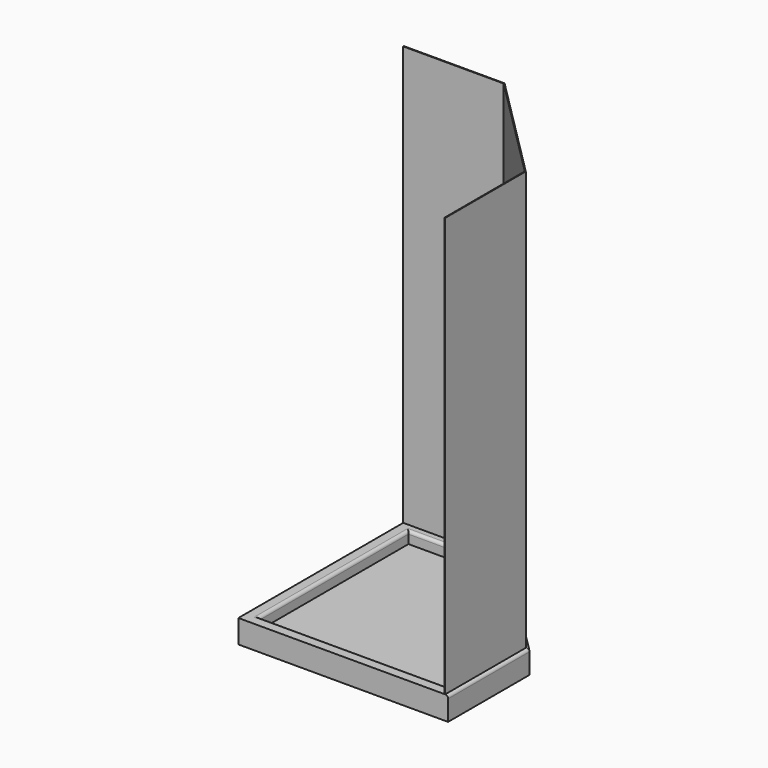
from build123d import *

# Parameters (mm, degrees)
F1_DEPTH     = 101.6
F2_T         = -50.8
F3_T1_DEPTH  = 508
F3_T3_DEPTH  = 728.0389529591
F3_T5_DEPTH  = 508
F3_T7_DEPTH  = 812.8
F3_T9_DEPTH  = 812.8
F3_T14_DEPTH = 685.954855022
F3_T20_DEPTH = 404.4079510314
F3_T25_DEPTH = 404.4079510314
F3_T31_DEPTH = 685.954855022
F3_T35_DEPTH = 404.4079510314
F3_T42_DEPTH = 404.4079510314
F3_T46_DEPTH = 685.954855022
F3_T53_DEPTH = 436.1579510314
F3_T57_DEPTH = 844.55
F3_T64_DEPTH = 844.55
F3_T68_DEPTH = 844.55
F3_T75_DEPTH = 844.55
F3_T79_DEPTH = 436.1579510314
F5_DEPTH     = 1828.8


# Not quite as in the source:
# - a fillet or chamfer that OpenCascade refuses, or shapes differently, is made with other operations: its cross-section is extruded or revolved along the edge and cut away or added


with BuildPart() as f1:
    # F0 (on Top) → F1 (new body)
    with BuildSketch(Plane.XY):
        Polygon((0, 914.4), (0, 0), (914.4, 0), (914.4, 444.5), (444.5, 914.4), align=None)
    extrude(amount=F1_DEPTH)

    # F2
    f2_openings = [f1.faces().sort_by_distance(p)[0] for p in [
        (411.47539, 411.47539, 101.6),
    ]]
    offset(amount=F2_T, openings=f2_openings)

    # F3: fillet of radius 12.7 on 11 edges, made by hand

    # F3_s2 → F3_t1 (cut)
    with BuildSketch(Plane.XZ.offset(-476.25)):
        with BuildLine():
            ThreePointArc((914.4, 88.9), (910.6802561211, 97.8802561211), (901.7, 101.6))
            Line((901.7, 101.6), (914.4, 101.6))
            Line((914.4, 101.6), (914.4, 88.9))
        make_face()
    extrude(amount=F3_T1_DEPTH, mode=Mode.SUBTRACT)

    # F3_s4 → F3_t3 (cut)
    with BuildSketch(Plane(origin=(257.4006403027, -257.4006403027, 0), x_dir=(0, 0, 1), z_dir=(-0.7071067812, 0.7071067812, 0))):
        with BuildLine():
            ThreePointArc((88.9, 960.8874049544), (97.8802561211, 957.1676610755), (101.6, 948.1874049544))
            Line((101.6, 948.1874049544), (101.6, 960.8874049544))
            Line((101.6, 960.8874049544), (88.9, 960.8874049544))
        make_face()
    extrude(amount=F3_T3_DEPTH, mode=Mode.SUBTRACT)

    # F3_s6 → F3_t5 (cut)
    with BuildSketch(Plane.YZ.offset(-31.75)):
        with BuildLine():
            ThreePointArc((914.4, 88.9), (910.6802561211, 97.8802561211), (901.7, 101.6))
            Line((901.7, 101.6), (914.4, 101.6))
            Line((914.4, 101.6), (914.4, 88.9))
        make_face()
    extrude(amount=F3_T5_DEPTH, mode=Mode.SUBTRACT)

    # F3_s8 → F3_t7 (cut)
    with BuildSketch(Plane.YZ.offset(50.8)):
        with BuildLine():
            ThreePointArc((38.1, 101.6), (47.0802561211, 97.8802561211), (50.8, 88.9))
            Line((50.8, 88.9), (50.8, 101.6))
            Line((50.8, 101.6), (38.1, 101.6))
        make_face()
    extrude(amount=F3_T7_DEPTH, mode=Mode.SUBTRACT)

    # F3_s10 → F3_t9 (cut)
    with BuildSketch(Plane.XZ.offset(-863.6)):
        with BuildLine():
            ThreePointArc((38.1, 101.6), (47.0802561211, 97.8802561211), (50.8, 88.9))
            Line((50.8, 88.9), (50.8, 101.6))
            Line((50.8, 101.6), (38.1, 101.6))
        make_face()
    extrude(amount=F3_T9_DEPTH, mode=Mode.SUBTRACT)


with BuildPart() as f3_tool12:
    # F3_s13 → F3_t14 (new body)
    with BuildSketch(Plane(origin=(242.5216647869, -242.5216647869, 0), x_dir=(0, 0, 1), z_dir=(-0.7071067812, 0.7071067812, 0))):
        with BuildLine():
            ThreePointArc((101.6, 922.7874049544), (97.8802561211, 913.8071488333), (88.9, 910.0874049544))
            Line((88.9, 910.0874049544), (101.6, 910.0874049544))
            Line((101.6, 910.0874049544), (101.6, 922.7874049544))
        make_face()
    extrude(amount=F3_T14_DEPTH)

    split(bisect_by=Plane.YZ.offset(863.6), keep=Keep.BOTTOM)

    split(bisect_by=Plane.XZ.offset(-863.6), keep=Keep.TOP)


with BuildPart() as f1_1:
    add(f1.part)

    # F3_t11: cut F3_tool12
    add(f3_tool12.part, mode=Mode.SUBTRACT)


with BuildPart() as f3_tool18:
    # F3_s19 → F3_t20 (new body)
    with BuildSketch(Plane.XZ.offset(-50.8)):
        with BuildLine():
            ThreePointArc((876.3, 101.6), (867.3197438789, 97.8802561211), (863.6, 88.9))
            Line((863.6, 88.9), (863.6, 101.6))
            Line((863.6, 101.6), (876.3, 101.6))
        make_face()
    extrude(amount=-F3_T20_DEPTH)

    split(bisect_by=Plane(origin=(643.5289755157, 643.5289755157, 0), x_dir=(0, 0, 1), z_dir=(-0.7071067812, -0.7071067812, 0)), keep=Keep.TOP)


with BuildPart() as f1_2:
    add(f1_1.part)

    # F3_t17: cut F3_tool18
    add(f3_tool18.part, mode=Mode.SUBTRACT)


with BuildPart() as f3_tool23:
    # F3_s24 → F3_t25 (new body)
    with BuildSketch(Plane.YZ.offset(455.2079510314)):
        with BuildLine():
            ThreePointArc((876.3, 101.6), (867.3197438789, 97.8802561211), (863.6, 88.9))
            Line((863.6, 88.9), (863.6, 101.6))
            Line((863.6, 101.6), (876.3, 101.6))
        make_face()
    extrude(amount=-F3_T25_DEPTH)

    split(bisect_by=Plane(origin=(643.5289755157, 643.5289755157, 0), x_dir=(0, 0, 1), z_dir=(-0.7071067812, -0.7071067812, 0)), keep=Keep.TOP)


with BuildPart() as f1_3:
    add(f1_2.part)

    # F3_t22: cut F3_tool23
    add(f3_tool23.part, mode=Mode.SUBTRACT)


with BuildPart() as f3_tool29:
    # F3_s30 → F3_t31 (new body)
    with BuildSketch(Plane(origin=(242.5216647869, -242.5216647869, 0), x_dir=(0, 0, 1), z_dir=(-0.7071067812, 0.7071067812, 0))):
        with BuildLine():
            ThreePointArc((101.6, 922.7874049544), (97.8802561211, 913.8071488333), (88.9, 910.0874049544))
            Line((88.9, 910.0874049544), (101.6, 910.0874049544))
            Line((101.6, 910.0874049544), (101.6, 922.7874049544))
        make_face()
    extrude(amount=F3_T31_DEPTH)

    split(bisect_by=Plane.YZ.offset(863.6), keep=Keep.TOP)


with BuildPart() as f3_tool33:
    # F3_s34 → F3_t35 (new body)
    with BuildSketch(Plane.XZ.offset(-50.8)):
        with BuildLine():
            ThreePointArc((876.3, 101.6), (867.3197438789, 97.8802561211), (863.6, 88.9))
            Line((863.6, 88.9), (863.6, 101.6))
            Line((863.6, 101.6), (876.3, 101.6))
        make_face()
    extrude(amount=-F3_T35_DEPTH)

    split(bisect_by=Plane(origin=(643.5289755157, 643.5289755157, 0), x_dir=(0, 0, 1), z_dir=(0.7071067812, 0.7071067812, 0)), keep=Keep.TOP)


with BuildPart() as f3_tool29_1:
    add(f3_tool29.part)

    # F3_t37: intersect F3_tool33
    add(f3_tool33.part, mode=Mode.INTERSECT)


with BuildPart() as f1_4:
    add(f1_3.part)

    # F3_t27: cut F3_tool29
    add(f3_tool29_1.part, mode=Mode.SUBTRACT)


with BuildPart() as f3_tool40:
    # F3_s41 → F3_t42 (new body)
    with BuildSketch(Plane.YZ.offset(455.2079510314)):
        with BuildLine():
            ThreePointArc((876.3, 101.6), (867.3197438789, 97.8802561211), (863.6, 88.9))
            Line((863.6, 88.9), (863.6, 101.6))
            Line((863.6, 101.6), (876.3, 101.6))
        make_face()
    extrude(amount=-F3_T42_DEPTH)

    split(bisect_by=Plane(origin=(643.5289755157, 643.5289755157, 0), x_dir=(0, 0, 1), z_dir=(0.7071067812, 0.7071067812, 0)), keep=Keep.TOP)


with BuildPart() as f3_tool44:
    # F3_s45 → F3_t46 (new body)
    with BuildSketch(Plane(origin=(242.5216647869, -242.5216647869, 0), x_dir=(0, 0, 1), z_dir=(-0.7071067812, 0.7071067812, 0))):
        with BuildLine():
            ThreePointArc((101.6, 922.7874049544), (97.8802561211, 913.8071488333), (88.9, 910.0874049544))
            Line((88.9, 910.0874049544), (101.6, 910.0874049544))
            Line((101.6, 910.0874049544), (101.6, 922.7874049544))
        make_face()
    extrude(amount=F3_T46_DEPTH)

    split(bisect_by=Plane.XZ.offset(-863.6), keep=Keep.BOTTOM)


with BuildPart() as f3_tool40_1:
    add(f3_tool40.part)

    # F3_t48: intersect F3_tool44
    add(f3_tool44.part, mode=Mode.INTERSECT)


with BuildPart() as f1_5:
    add(f1_4.part)

    # F3_t38: cut F3_tool40
    add(f3_tool40_1.part, mode=Mode.SUBTRACT)


with BuildPart() as f3_tool51:
    # F3_s52 → F3_t53 (new body)
    with BuildSketch(Plane.XZ.offset(-19.05)):
        with BuildLine():
            ThreePointArc((876.3, 101.6), (867.3197438789, 97.8802561211), (863.6, 88.9))
            Line((863.6, 88.9), (863.6, 101.6))
            Line((863.6, 101.6), (876.3, 101.6))
        make_face()
    extrude(amount=-F3_T53_DEPTH)

    split(bisect_by=Plane.XZ.offset(-50.8), keep=Keep.TOP)


with BuildPart() as f3_tool55:
    # F3_s56 → F3_t57 (new body)
    with BuildSketch(Plane.YZ.offset(50.8)):
        with BuildLine():
            ThreePointArc((38.1, 101.6), (47.0802561211, 97.8802561211), (50.8, 88.9))
            Line((50.8, 88.9), (50.8, 101.6))
            Line((50.8, 101.6), (38.1, 101.6))
        make_face()
    extrude(amount=F3_T57_DEPTH)

    split(bisect_by=Plane.YZ.offset(863.6), keep=Keep.TOP)


with BuildPart() as f3_tool51_1:
    add(f3_tool51.part)

    # F3_t59: intersect F3_tool55
    add(f3_tool55.part, mode=Mode.INTERSECT)


with BuildPart() as f1_6:
    add(f1_5.part)

    # F3_t49: cut F3_tool51
    add(f3_tool51_1.part, mode=Mode.SUBTRACT)


with BuildPart() as f3_tool62:
    # F3_s63 → F3_t64 (new body)
    with BuildSketch(Plane.XZ.offset(-863.6)):
        with BuildLine():
            ThreePointArc((38.1, 101.6), (47.0802561211, 97.8802561211), (50.8, 88.9))
            Line((50.8, 88.9), (50.8, 101.6))
            Line((50.8, 101.6), (38.1, 101.6))
        make_face()
    extrude(amount=F3_T64_DEPTH)

    split(bisect_by=Plane.XZ.offset(-50.8), keep=Keep.TOP)


with BuildPart() as f3_tool66:
    # F3_s67 → F3_t68 (new body)
    with BuildSketch(Plane.YZ.offset(19.05)):
        with BuildLine():
            ThreePointArc((38.1, 101.6), (47.0802561211, 97.8802561211), (50.8, 88.9))
            Line((50.8, 88.9), (50.8, 101.6))
            Line((50.8, 101.6), (38.1, 101.6))
        make_face()
    extrude(amount=F3_T68_DEPTH)

    split(bisect_by=Plane.YZ.offset(50.8), keep=Keep.BOTTOM)


with BuildPart() as f3_tool62_1:
    add(f3_tool62.part)

    # F3_t70: intersect F3_tool66
    add(f3_tool66.part, mode=Mode.INTERSECT)


with BuildPart() as f1_7:
    add(f1_6.part)

    # F3_t60: cut F3_tool62
    add(f3_tool62_1.part, mode=Mode.SUBTRACT)


with BuildPart() as f3_tool73:
    # F3_s74 → F3_t75 (new body)
    with BuildSketch(Plane.XZ.offset(-895.35)):
        with BuildLine():
            ThreePointArc((38.1, 101.6), (47.0802561211, 97.8802561211), (50.8, 88.9))
            Line((50.8, 88.9), (50.8, 101.6))
            Line((50.8, 101.6), (38.1, 101.6))
        make_face()
    extrude(amount=F3_T75_DEPTH)

    split(bisect_by=Plane.XZ.offset(-863.6), keep=Keep.BOTTOM)


with BuildPart() as f3_tool77:
    # F3_s78 → F3_t79 (new body)
    with BuildSketch(Plane.YZ.offset(455.2079510314)):
        with BuildLine():
            ThreePointArc((876.3, 101.6), (867.3197438789, 97.8802561211), (863.6, 88.9))
            Line((863.6, 88.9), (863.6, 101.6))
            Line((863.6, 101.6), (876.3, 101.6))
        make_face()
    extrude(amount=-F3_T79_DEPTH)

    split(bisect_by=Plane.YZ.offset(50.8), keep=Keep.BOTTOM)


with BuildPart() as f3_tool73_1:
    add(f3_tool73.part)

    # F3_t81: intersect F3_tool77
    add(f3_tool77.part, mode=Mode.INTERSECT)


with BuildPart() as f1_8:
    add(f1_7.part)

    # F3_t71: cut F3_tool73
    add(f3_tool73_1.part, mode=Mode.SUBTRACT)


with BuildPart() as f5:
    # F4 (on face) → F5 (new body)
    with BuildSketch(Plane.XY.offset(101.6)):
        Polygon((898.525, 0), (901.7, 0), (901.7, 439.2394877579), (439.2394877579, 901.7), (0, 901.7), (0, 898.525), (437.9243596973, 898.525), (898.525, 437.9243596973), align=None)
    extrude(amount=F5_DEPTH)


solid = Compound([f1_8.part, f5.part])
